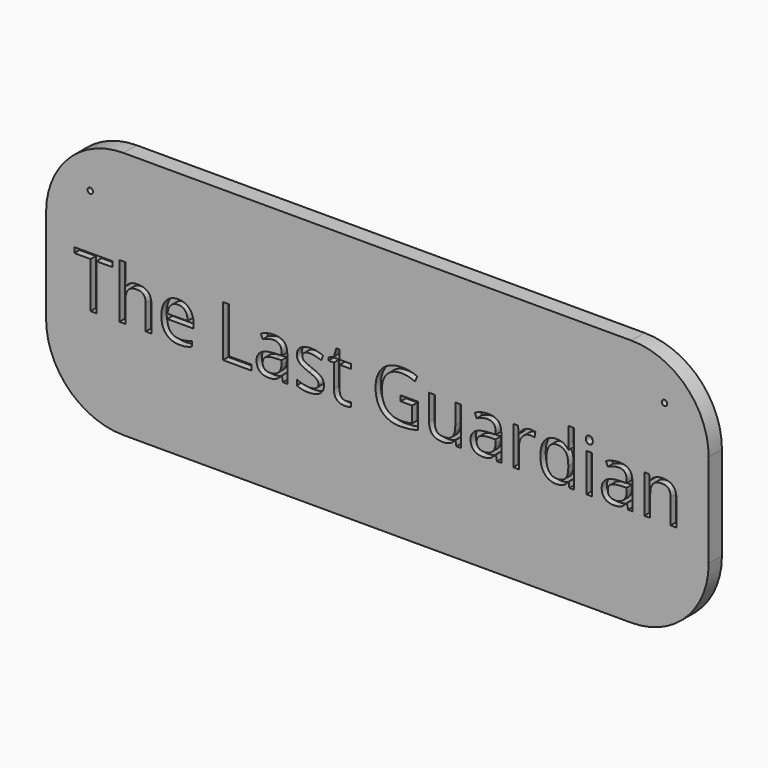
from build123d import *

# Parameters (mm, degrees)
F0_W         = 600
F0_H         = 225
F1_DEPTH     = 15
F3_R         = 70
F2_TEXT_SIZE = 64.8656617403
F4_DEPTH     = 6
F5_R         = 2.5
F6_DEPTH     = 25


# Not quite as in the source:
# - Text() gives the source's letters only with a copy of the font that has no kerning and outlines rounded to 1/6400 em; it was checked with that copy


with BuildPart() as f1:
    # F0 (on Front) → F1 (new body)
    with BuildSketch(Plane.XZ):
        Rectangle(F0_W, F0_H)
    extrude(amount=F1_DEPTH)

    # F3
    f3_edges = [f1.edges().sort_by_distance(p)[0] for p in [
        (300, -7.5, 112.5),
        (300, -7.5, -112.5),
        (-300, -7.5, -112.5),
        (-300, -7.5, 112.5),
    ]]
    fillet(f3_edges, radius=F3_R)

    # F2 (on face) → F4 (cut)
    with BuildSketch(Plane.XZ.offset(15)):
        with Locations((-275.0000221314, -23.3515835827)):
            Text('The Last Guardian', F2_TEXT_SIZE, font='Open Sans', text_align=(TextAlign.LEFT, TextAlign.BOTTOM))
    extrude(amount=-F4_DEPTH, mode=Mode.SUBTRACT)

    # F5 (on face) → F6 (cut)
    with BuildSketch(Plane.XZ.offset(15)):
        with Locations((-260, 72.5)):
            Circle(F5_R)
        with Locations((260, 72.5)):
            Circle(F5_R)
    extrude(amount=-F6_DEPTH, mode=Mode.SUBTRACT)


with BuildPart() as f7_1:
    # F7: copy of F1
    add(f1.part)


solid = Compound([f1.part, f7_1.part])
